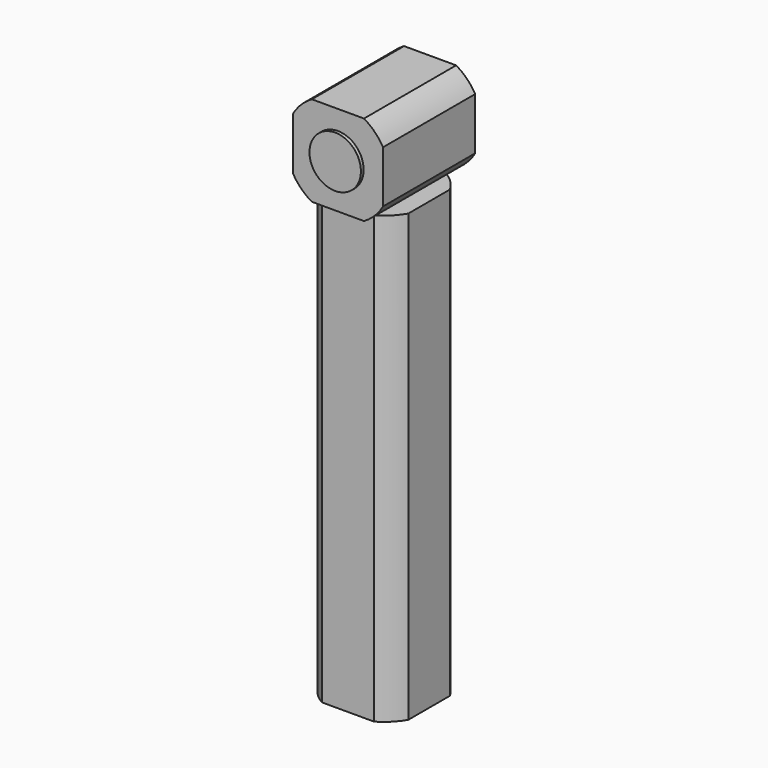
from build123d import *

# Parameters (mm, degrees)
F0_R          = 37.5
F1_DEPTH      = 84
F1_DEPTH_BACK = 84
F2_DEPTH      = 89
F2_DEPTH_BACK = 89
F3_W          = 76
F3_H          = 131.6358613752
F3_R          = 37.5
F4_DEPTH      = 650


with BuildPart() as f1:
    # F0 (on Front) → F1 (new body, two sides)
    with BuildSketch(Plane.XZ) as f1_sk:
        with BuildLine():
            Line((-65.8179306876, 38), (-65.8179306876, -38))
            ThreePointArc((-65.8179306876, -38), (-53.7401153702, -53.7401153702), (-38, -65.8179306876))
            Line((-38, -65.8179306876), (38, -65.8179306876))
            ThreePointArc((38, -65.8179306876), (53.7401153702, -53.7401153702), (65.8179306876, -38))
            Line((65.8179306876, -38), (65.8179306876, 38))
            ThreePointArc((65.8179306876, 38), (53.7401153702, 53.7401153702), (38, 65.8179306876))
            Line((38, 65.8179306876), (-38, 65.8179306876))
            ThreePointArc((-38, 65.8179306876), (-53.7401153702, 53.7401153702), (-65.8179306876, 38))
        make_face()
        Circle(F0_R, mode=Mode.SUBTRACT)
        Circle(F0_R)
    extrude(amount=F1_DEPTH)
    extrude(f1_sk.sketch, amount=-F1_DEPTH_BACK)

    # F0 (on Front) → F2 (join, two sides)
    with BuildSketch(Plane.XZ) as f2_sk:
        Circle(F0_R)
    extrude(amount=F2_DEPTH)
    extrude(f2_sk.sketch, amount=-F2_DEPTH_BACK)

    # F3 (on face) → F4 (join)
    with BuildSketch(Plane(origin=(0, 0, -65.8179306876), x_dir=(1, 0, 0), z_dir=(0, 0, -1))):
        Rectangle(F3_W, F3_H)
        Circle(F3_R, mode=Mode.SUBTRACT)
        Circle(F3_R)
        with BuildLine():
            Line((-65.8179306876, 38), (-65.8179306876, -38))
            ThreePointArc((-65.8179306876, -38), (-53.7401153702, -53.7401153702), (-38, -65.8179306876))
            Line((-38, -65.8179306876), (-38, 65.8179306876))
            ThreePointArc((-38, 65.8179306876), (-53.7401153702, 53.7401153702), (-65.8179306876, 38))
        make_face()
        with BuildLine():
            Line((38, 65.8179306876), (38, -65.8179306876))
            ThreePointArc((38, -65.8179306876), (53.7401153702, -53.7401153702), (65.8179306876, -38))
            Line((65.8179306876, -38), (65.8179306876, 38))
            ThreePointArc((65.8179306876, 38), (53.7401153702, 53.7401153702), (38, 65.8179306876))
        make_face()
    extrude(amount=F4_DEPTH)


solid = f1.part
